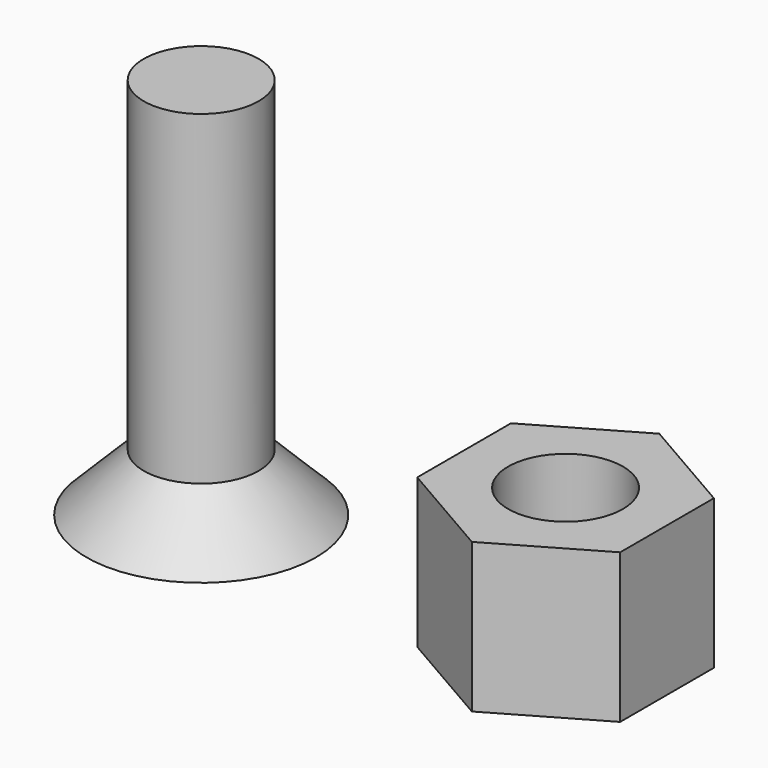
from build123d import *

# Parameters (mm, degrees)
F0_R     = 1.5
F1_DEPTH = 10
F0_R_2   = 3
F2_DEPTH = 1.5
F3_SIZE  = 1.49999
F4_DEPTH = 3.9


# Not quite as in the source:
# - a fillet or chamfer is up to 0.001 mm smaller than in the source, because OpenCascade refuses the exact size


with BuildPart() as f1:
    # F0 (on Top) → F1 (new body)
    with BuildSketch(Plane.XY):
        with Locations((-21.6073635966, 27.3428875953)):
            Circle(F0_R)
    extrude(amount=F1_DEPTH)

    # F0 (on Top) → F2 (join)
    with BuildSketch(Plane.XY):
        with Locations((-21.6073635966, 27.3428875953)):
            Circle(F0_R_2)
        with Locations((-21.6073635966, 27.3428875953)):
            Circle(F0_R, mode=Mode.SUBTRACT)
    extrude(amount=F2_DEPTH)

    # F3 (size 1.5 in the source; OpenCascade refuses exactly that, so slightly less here)
    f3_edges = [f1.edges().sort_by_distance(p)[0] for p in [
        (-24.607364, 27.342888, 1.5),
    ]]
    chamfer(f3_edges, length=F3_SIZE)


with BuildPart() as f4:
    # F0 (on Top) → F4 (new body)
    with BuildSketch(Plane.XY):
        Polygon((-9.2233226543, 25.5416321092), (-9.2233226543, 28.6015885359), (-11.8733226543, 30.1315667493), (-14.5233226543, 28.6015885359), (-14.5233226543, 25.5416321092), (-11.8733226543, 24.0116538959), align=None)
        with Locations((-11.8733226543, 27.0716103226)):
            Circle(F0_R, mode=Mode.SUBTRACT)
    extrude(amount=F4_DEPTH)


solid = Compound([f1.part, f4.part])
